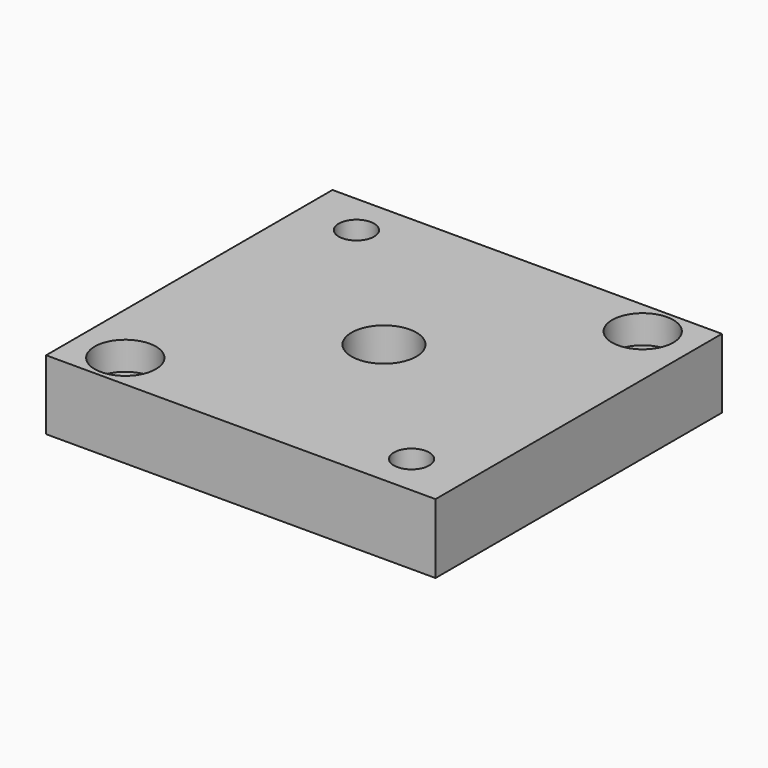
from build123d import *

# Parameters (mm, degrees)
F0_W      = 42
F0_H      = 38.608
F1_DEPTH  = 7.493
F2_R      = 1.905
F3_DEPTH  = 7.494
F4_R      = 1.905
F5_DEPTH  = 25.4
F6_R      = 3.302
F6_R_2    = 1.905
F7_DEPTH  = 3.048
F8_R      = 3.5
F9_DEPTH  = 7.494
F10_R     = 12
F11_DEPTH = 3
F13_DEPTH = 3.81


with BuildPart() as f1:
    # F0 (on Top) → F1 (new body)
    with BuildSketch(Plane.XY):
        Rectangle(F0_W, F0_H)
    extrude(amount=F1_DEPTH)

    # F2 (on face) → F3 (cut, through all)
    with BuildSketch(Plane.XY.offset(7.493)):
        with Locations((-14.8492424049, 14.8492424049)):
            Circle(F2_R)
        with Locations((14.8492424049, -14.8492424049)):
            Circle(F2_R)
    extrude(amount=-F3_DEPTH, mode=Mode.SUBTRACT)

    # F4 (on face) → F5 (cut)
    with BuildSketch(Plane.XY.offset(7.493)):
        with Locations((15.5, 15.5)):
            Circle(F4_R)
        with Locations((-15.5, -15.5)):
            Circle(F4_R)
    extrude(amount=-F5_DEPTH, mode=Mode.SUBTRACT)

    # F6 (on face) → F7 (cut)
    with BuildSketch(Plane.XY.offset(7.493)):
        with Locations((15.5, 15.5)):
            Circle(F6_R)
        with Locations((15.5, 15.5)):
            Circle(F6_R_2, mode=Mode.SUBTRACT)
        with Locations((-15.5, -15.5)):
            Circle(F6_R)
        with Locations((-15.5, -15.5)):
            Circle(F6_R_2, mode=Mode.SUBTRACT)
        with Locations((15.5, 15.5)):
            Circle(F6_R_2)
        with Locations((-15.5, -15.5)):
            Circle(F6_R_2)
    extrude(amount=-F7_DEPTH, mode=Mode.SUBTRACT)

    # F8 (on face) → F9 (cut, through all)
    with BuildSketch(Plane.XY.offset(7.493)):
        Circle(F8_R)
    extrude(amount=-F9_DEPTH, mode=Mode.SUBTRACT)

    # F10 (on face) → F11 (cut)
    with BuildSketch(Plane(origin=(0, 0, 0), x_dir=(1, 0, 0), z_dir=(0, 0, -1))):
        Circle(F10_R)
    extrude(amount=-F11_DEPTH, mode=Mode.SUBTRACT)

    # F12 (on face) → F13 (cut)
    with BuildSketch(Plane(origin=(0, 0, 0), x_dir=(1, 0, 0), z_dir=(0, 0, -1))):
        Polygon((18.2782424049, 12.8695083319), (18.2782424049, 16.828976478), (14.8492424049, 18.808710551), (11.4202424049, 16.828976478), (11.4202424049, 12.8695083319), (14.8492424049, 10.8897742588), align=None)
        Polygon((-11.4202424049, -16.828976478), (-11.4202424049, -12.8695083319), (-14.8492424049, -10.8897742588), (-18.2782424049, -12.8695083319), (-18.2782424049, -16.828976478), (-14.8492424049, -18.808710551), align=None)
    extrude(amount=-F13_DEPTH, mode=Mode.SUBTRACT)


solid = f1.part
